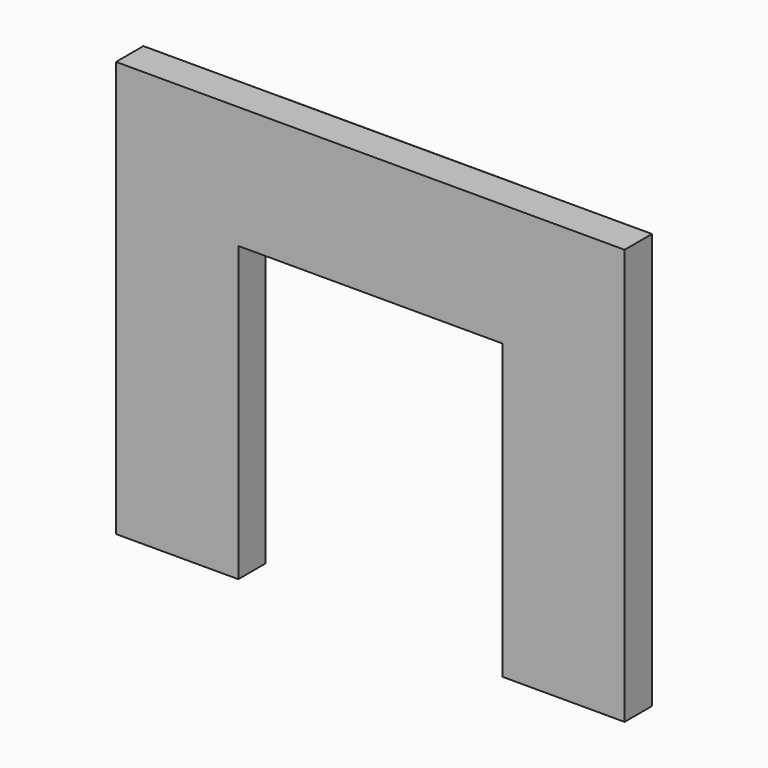
from build123d import *

# Parameters (mm, degrees)
F1_DEPTH = 1.778
F3_DEPTH = 6.35
F4_R     = 0.25399


# Not quite as in the source:
# - a fillet or chamfer is up to 0.001 mm smaller than in the source, because OpenCascade refuses the exact size


with BuildPart() as f1:
    # F0 (on Front) → F1 (new body)
    with BuildSketch(Plane.XZ):
        Polygon((-6.858, -10.8697404989), (-6.858, 4.3702595011), (0, 4.3702595011), (6.858, 4.3702595011), (6.858, -10.8697404989), (13.208, -10.8697404989), (13.208, 10.7202595011), (-13.208, 10.7202595011), (-13.208, -10.8697404989), align=None)
    extrude(amount=F1_DEPTH)

    # F2 (on Right) → F3 (join, symmetric)
    with BuildSketch(Plane.YZ):
        with BuildLine():
            ThreePointArc((0.254, 10.3265595011), (0.1849893869, 10.5608220088), (0, 10.7202595011))
            Line((0, 10.7202595011), (0, 10.3265595011))
            Line((0, 10.3265595011), (0.254, 10.3265595011))
        make_face()
        with BuildLine():
            Line((0.254, 10.3265595011), (0, 10.3265595011))
            Line((0, 10.3265595011), (0, 9.9328595011))
            ThreePointArc((0, 9.9328595011), (0.1849893869, 10.0922969934), (0.254, 10.3265595011))
        make_face()
    extrude(amount=F3_DEPTH, both=True)

    # F4 (radius 0.254 in the source; OpenCascade refuses exactly that, so slightly less here)
    f4_edges = [f1.edges().sort_by_distance(p)[0] for p in [
        (-6.35, 0.254, 10.32656),
        (6.35, 0.254, 10.32656),
    ]]
    fillet(f4_edges, radius=F4_R)


solid = f1.part
